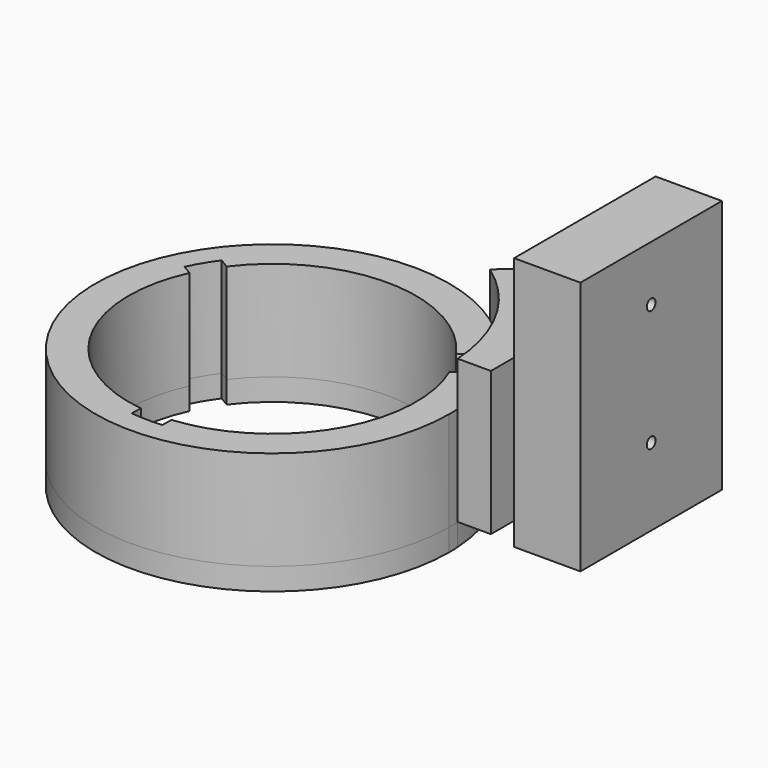
from build123d import *
from build123d import SkipClean  # not in build123d's __all__

# Parameters (mm, degrees)
F1_DEPTH = 9
F2_DEPTH = 13
F4_DEPTH = 2.5
F6_DEPTH = 6
F7_R     = 0.5
F8_DEPTH = 10
F9_DEPTH = 2


with BuildPart() as f1:
    # F0 (on Top) → F1 (new body)
    with BuildSketch(Plane.XY):
        with BuildLine():
            ThreePointArc((9.210061901, 13.0833772314), (-14.201425816, -7.3701767138), (16, 0))
            ThreePointArc((16, 0), (15.9921779437, 0.5002445588), (15.9687194227, 1))
            ThreePointArc((15.9687194227, 1), (13.964052369, 7.8105852172), (9.210061901, 13.0833772314))
        make_face()
        with BuildLine():
            Line((10.5963823009, 7.5310478775), (11.473873387, 8.0218594789))
            ThreePointArc((11.473873387, 8.0218594789), (12.2185458229, 6.834262065), (12.8407258, 5.5781503143))
            Line((12.8407258, 5.5781503143), (11.9632347139, 5.0873387129))
            ThreePointArc((11.9632347139, 5.0873387129), (11.1687805133, -6.6526943298), (1.2238876286, -12.9422601995))
            Line((1.2238876286, -12.9422601995), (1.2101974008, -13.9475955724))
            ThreePointArc((1.2101974008, -13.9475955724), (-0.190628347, -13.9987021125), (-1.5895430217, -13.909469903))
            Line((-1.5895430217, -13.909469903), (-1.5758527939, -12.9041345301))
            ThreePointArc((-1.5758527939, -12.9041345301), (-11.3457925498, -6.346100489), (-11.8202699295, 5.4112123221))
            Line((-11.8202699295, 5.4112123221), (-12.6840707878, 5.9257360935))
            ThreePointArc((-12.6840707878, 5.9257360935), (-12.0279174759, 7.1644400474), (-11.2511827783, 8.3313195887))
            Line((-11.2511827783, 8.3313195887), (-10.38738192, 7.8167958172))
            ThreePointArc((-10.38738192, 7.8167958172), (0.1770120365, 12.9987948187), (10.5963823009, 7.5310478775))
        make_face(mode=Mode.SUBTRACT)
        with BuildLine():
            ThreePointArc((9.210061901, 13.0833772314), (13.964052369, 7.8105852172), (15.9687194227, 1))
            Line((15.9687194227, 1), (18.9687194227, 1))
            Line((18.9687194227, 1), (18.9687194227, 16))
            Line((18.9687194227, 16), (12.4687194227, 16))
            Line((12.4687194227, 16), (9.210061901, 13.0833772314))
        make_face()
    extrude(amount=F1_DEPTH)

    # F0 (on Top) → F2 (join)
    with BuildSketch(Plane.XY):
        with BuildLine():
            ThreePointArc((9.210061901, 13.0833772314), (13.964052369, 7.8105852172), (15.9687194227, 1))
            Line((15.9687194227, 1), (18.9687194227, 1))
            Line((18.9687194227, 1), (18.9687194227, 16))
            Line((18.9687194227, 16), (12.4687194227, 16))
            Line((12.4687194227, 16), (9.210061901, 13.0833772314))
        make_face()
    extrude(amount=F2_DEPTH)

    # F3 (on face) → F4 (join)
    with BuildSketch(Plane.YZ.offset(18.9687194227)):
        with BuildLine():
            Line((3.85, 8.35), (3.85, 0))
            Line((3.85, 0), (13.15, 0))
            Line((13.15, 0), (13.15, 8.35))
            ThreePointArc((13.15, 8.35), (11.7880465325, 11.6380465325), (8.5, 13))
            ThreePointArc((8.5, 13), (5.2119534675, 11.6380465325), (3.85, 8.35))
        make_face()
    extrude(amount=F4_DEPTH)

    # F5 (on face) → F6 (join)
    with BuildSketch(Plane.YZ.offset(21.4687194227)):
        with BuildLine():
            Line((0.5, 23), (0.5, 0))
            Line((0.5, 0), (3.85, 0))
            Line((3.85, 0), (3.85, 8.35))
            ThreePointArc((3.85, 8.35), (8.5, 13), (13.15, 8.35))
            Line((13.15, 8.35), (13.15, 0))
            Line((13.15, 0), (16.5, 0))
            Line((16.5, 0), (16.5, 23))
            Line((16.5, 23), (0.5, 23))
        make_face()
        with BuildLine():
            Line((3.85, 8.35), (3.85, 0))
            Line((3.85, 0), (13.15, 0))
            Line((13.15, 0), (13.15, 8.35))
            ThreePointArc((13.15, 8.35), (8.5, 13), (3.85, 8.35))
        make_face()
    extrude(amount=F6_DEPTH)

    # F7 (on face) → F8 (cut)
    with BuildSketch(Plane.YZ.offset(27.4687194227)):
        with Locations((8.5, 7)):
            Circle(F7_R)
        with Locations((8.5, 18)):
            Circle(F7_R)
    extrude(amount=-F8_DEPTH, mode=Mode.SUBTRACT)

    # F0 (on Top) → F9 (join)
    with BuildSketch(Plane.XY):
        with BuildLine():
            ThreePointArc((9.210061901, 13.0833772314), (-14.201425816, -7.3701767138), (16, 0))
            ThreePointArc((16, 0), (15.9921779437, 0.5002445588), (15.9687194227, 1))
            ThreePointArc((15.9687194227, 1), (13.964052369, 7.8105852172), (9.210061901, 13.0833772314))
        make_face()
        with BuildLine():
            Line((10.5963823009, 7.5310478775), (11.473873387, 8.0218594789))
            ThreePointArc((11.473873387, 8.0218594789), (12.2185458229, 6.834262065), (12.8407258, 5.5781503143))
            Line((12.8407258, 5.5781503143), (11.9632347139, 5.0873387129))
            ThreePointArc((11.9632347139, 5.0873387129), (11.1687805133, -6.6526943298), (1.2238876286, -12.9422601995))
            Line((1.2238876286, -12.9422601995), (1.2101974008, -13.9475955724))
            ThreePointArc((1.2101974008, -13.9475955724), (-0.190628347, -13.9987021125), (-1.5895430217, -13.909469903))
            Line((-1.5895430217, -13.909469903), (-1.5758527939, -12.9041345301))
            ThreePointArc((-1.5758527939, -12.9041345301), (-11.3457925498, -6.346100489), (-11.8202699295, 5.4112123221))
            Line((-11.8202699295, 5.4112123221), (-12.6840707878, 5.9257360935))
            ThreePointArc((-12.6840707878, 5.9257360935), (-12.0279174759, 7.1644400474), (-11.2511827783, 8.3313195887))
            Line((-11.2511827783, 8.3313195887), (-10.38738192, 7.8167958172))
            ThreePointArc((-10.38738192, 7.8167958172), (0.1770120365, 12.9987948187), (10.5963823009, 7.5310478775))
        make_face(mode=Mode.SUBTRACT)
    with SkipClean():  # cleaning this boolean's faces spoils the solid; the shape is the same uncleaned
        extrude(amount=-F9_DEPTH)


solid = f1.part
